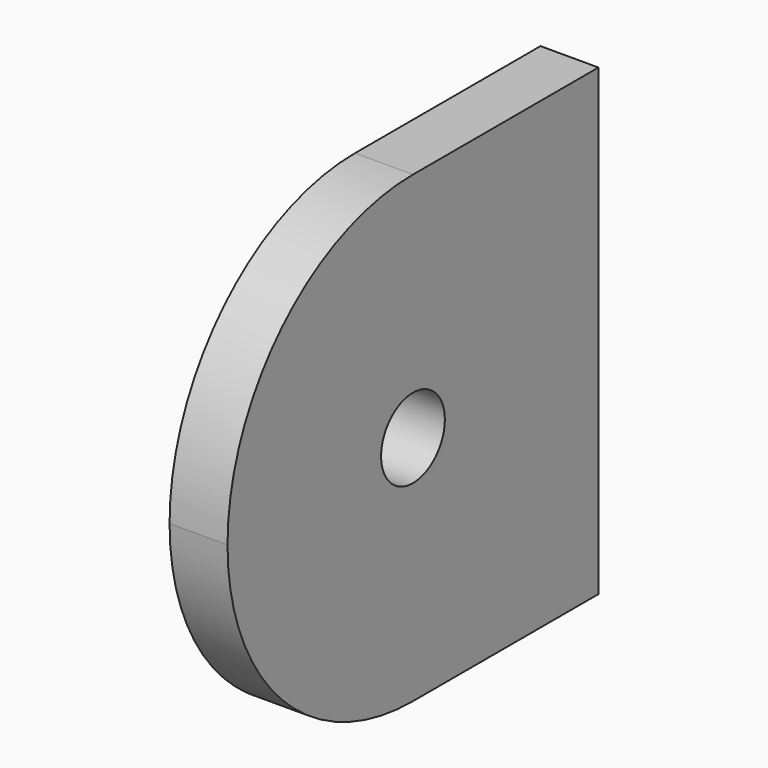
from build123d import *

# Parameters (mm, degrees)
F0_W     = 101.6
F0_H     = 101.6
F1_DEPTH = 6.35
F2_R     = 50.79999
F3_R     = 8.73125
F4_DEPTH = 25.4


# Not quite as in the source:
# - a fillet or chamfer is up to 0.001 mm smaller than in the source, because OpenCascade refuses the exact size


with BuildPart() as f1:
    # F0 (on Right) → F1 (new body, symmetric)
    with BuildSketch(Plane.YZ):
        with Locations((-50.8, 50.8)):
            Rectangle(F0_W, F0_H)
    extrude(amount=F1_DEPTH, both=True)

    # F2 (radius 50.8 in the source; OpenCascade refuses exactly that, so slightly less here)
    f2_edges = [f1.edges().sort_by_distance(p)[0] for p in [
        (0, -101.6, 101.6),
        (0, -101.6, 0),
    ]]
    fillet(f2_edges, radius=F2_R)

    # F3 (on face) → F4 (cut)
    with BuildSketch(Plane.YZ.offset(6.35)):
        with Locations((-50.8, 50.8)):
            Circle(F3_R)
    extrude(amount=-F4_DEPTH, mode=Mode.SUBTRACT)


solid = f1.part
